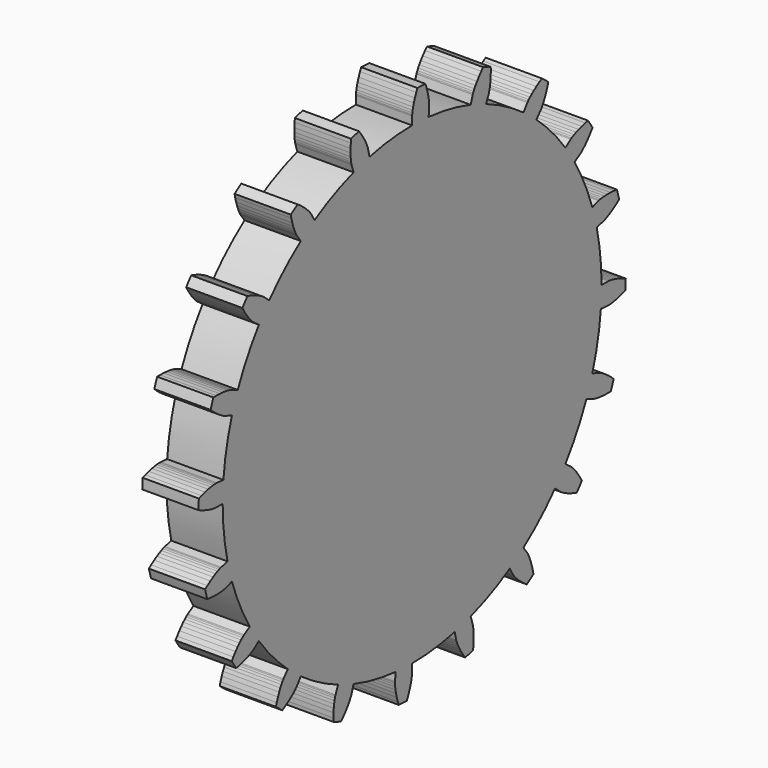
from build123d import *

# Parameters (mm, degrees)
F2_DEPTH = 6.35


# Not quite as in the source:
# - a variable given as a bare number and used for a length is read in inches; the dataset says mm whatever the document's units were


with BuildPart() as f2:
    # F1 (on Right) → F2 (new body)
    with BuildSketch(Plane.YZ):
        with BuildLine():
            ThreePointArc((26.6365153387, -2.330393128), (26.7128135988, -1.1663066295), (26.7382625, 0))
            ThreePointArc((26.7382625, 0), (26.5663850897, 3.0268572456), (26.0529625644, 6.0148003407))
            ThreePointArc((26.0529625644, 6.0148003407), (25.7658040109, 7.1454898497), (25.429598785, 8.2625775126))
            ThreePointArc((25.429598785, 8.2625775126), (24.3307833255, 11.0881767791), (22.9191642926, 13.7712232444))
            ThreePointArc((22.9191642926, 13.7712232444), (22.2966580055, 14.7578359967), (21.6317087626, 15.7163563694))
            ThreePointArc((21.6317087626, 15.7163563694), (19.7135149669, 18.0641083137), (17.5418785326, 20.1796228673))
            ThreePointArc((17.5418785326, 20.1796228673), (16.6449597645, 20.9255823326), (15.7163563694, 21.6317087626))
            ThreePointArc((15.7163563694, 21.6317087626), (13.1665504112, 23.2717990664), (10.4474714805, 24.6127004041))
            ThreePointArc((10.4474714805, 24.6127004041), (9.3639368896, 25.0449868726), (8.2625775126, 25.429598785))
            ThreePointArc((8.2625775126, 25.429598785), (5.3307521645, 26.2014839824), (2.330393128, 26.6365153387))
            ThreePointArc((2.330393128, 26.6365153387), (1.1663066295, 26.7128135988), (0, 26.7382625))
            ThreePointArc((0, 26.7382625), (-3.0268572456, 26.5663850897), (-6.0148003407, 26.0529625644))
            ThreePointArc((-6.0148003407, 26.0529625644), (-7.1454898497, 25.7658040109), (-8.2625775126, 25.429598785))
            ThreePointArc((-8.2625775126, 25.429598785), (-11.0881767791, 24.3307833255), (-13.7712232444, 22.9191642926))
            ThreePointArc((-13.7712232444, 22.9191642926), (-14.7578359967, 22.2966580055), (-15.7163563694, 21.6317087626))
            ThreePointArc((-15.7163563694, 21.6317087626), (-18.0641083137, 19.7135149669), (-20.1796228673, 17.5418785326))
            ThreePointArc((-20.1796228673, 17.5418785326), (-20.9255823326, 16.6449597645), (-21.6317087626, 15.7163563694))
            ThreePointArc((-21.6317087626, 15.7163563694), (-23.2717990664, 13.1665504112), (-24.6127004041, 10.4474714805))
            ThreePointArc((-24.6127004041, 10.4474714805), (-25.0449868726, 9.3639368896), (-25.429598785, 8.2625775126))
            ThreePointArc((-25.429598785, 8.2625775126), (-26.2014839824, 5.3307521645), (-26.6365153387, 2.330393128))
            ThreePointArc((-26.6365153387, 2.330393128), (-26.7128135988, 1.1663066295), (-26.7382625, 0))
            ThreePointArc((-26.7382625, 0), (-26.5663850897, -3.0268572456), (-26.0529625644, -6.0148003407))
            ThreePointArc((-26.0529625644, -6.0148003407), (-25.7658040109, -7.1454898497), (-25.429598785, -8.2625775126))
            ThreePointArc((-25.429598785, -8.2625775126), (-24.3307833255, -11.0881767791), (-22.9191642926, -13.7712232444))
            ThreePointArc((-22.9191642926, -13.7712232444), (-22.2966580055, -14.7578359967), (-21.6317087626, -15.7163563694))
            ThreePointArc((-21.6317087626, -15.7163563694), (-19.7135149669, -18.0641083137), (-17.5418785326, -20.1796228673))
            ThreePointArc((-17.5418785326, -20.1796228673), (-16.6449597645, -20.9255823326), (-15.7163563694, -21.6317087626))
            ThreePointArc((-15.7163563694, -21.6317087626), (-13.1665504112, -23.2717990664), (-10.4474714805, -24.6127004041))
            ThreePointArc((-10.4474714805, -24.6127004041), (-9.3639368896, -25.0449868726), (-8.2625775126, -25.429598785))
            ThreePointArc((-8.2625775126, -25.429598785), (-5.3307521645, -26.2014839824), (-2.330393128, -26.6365153387))
            ThreePointArc((-2.330393128, -26.6365153387), (-1.1663066295, -26.7128135988), (0, -26.7382625))
            ThreePointArc((0, -26.7382625), (3.0268572456, -26.5663850897), (6.0148003407, -26.0529625644))
            ThreePointArc((6.0148003407, -26.0529625644), (7.1454898497, -25.7658040109), (8.2625775126, -25.429598785))
            ThreePointArc((8.2625775126, -25.429598785), (11.0881767791, -24.3307833255), (13.7712232444, -22.9191642926))
            ThreePointArc((13.7712232444, -22.9191642926), (14.7578359967, -22.2966580055), (15.7163563694, -21.6317087626))
            ThreePointArc((15.7163563694, -21.6317087626), (18.0641083137, -19.7135149669), (20.1796228673, -17.5418785326))
            ThreePointArc((20.1796228673, -17.5418785326), (20.9255823326, -16.6449597645), (21.6317087626, -15.7163563694))
            ThreePointArc((21.6317087626, -15.7163563694), (23.2717990664, -13.1665504112), (24.6127004041, -10.4474714805))
            ThreePointArc((24.6127004041, -10.4474714805), (25.0449868726, -9.3639368896), (25.429598785, -8.2625775126))
            ThreePointArc((25.429598785, -8.2625775126), (26.2014839824, -5.3307521645), (26.6365153387, -2.330393128))
        make_face()
        with BuildLine():
            Line((-26.3108062145, -8.5488991629), (-25.429598785, -8.2625775126))
            ThreePointArc((-25.429598785, -8.2625775126), (-25.7658040109, -7.1454898497), (-26.0529625644, -6.0148003407))
            Line((-26.0529625644, -6.0148003407), (-26.9557713096, -6.2232301626))
            Line((-26.9557713096, -6.2232301626), (-26.9891857357, -6.2321271956))
            Line((-26.9891857357, -6.2321271956), (-27.088141079, -6.2632448013))
            Line((-27.088141079, -6.2632448013), (-27.250334693, -6.3231051855))
            Line((-27.250334693, -6.3231051855), (-27.4729785748, -6.4180477409))
            Line((-27.4729785748, -6.4180477409), (-27.7528122899, -6.5541969827))
            Line((-27.7528122899, -6.5541969827), (-28.0861178795, -6.73743134))
            Line((-28.0861178795, -6.73743134), (-28.4687366983, -6.9733529183))
            Line((-28.4687366983, -6.9733529183), (-28.8960881212, -7.2672583507))
            Line((-28.8960881212, -7.2672583507), (-29.2128054383, -7.5092213093))
            ThreePointArc((-29.2128054383, -7.5092213093), (-29.0655035449, -8.0605775185), (-28.9077964707, -8.6090481156))
            Line((-28.9077964707, -8.6090481156), (-28.5116966065, -8.6533293744))
            Line((-28.5116966065, -8.6533293744), (-27.9940124528, -8.6851532464))
            Line((-27.9940124528, -8.6851532464), (-27.5445355172, -8.690314249))
            Line((-27.5445355172, -8.690314249), (-27.164464194, -8.6757116792))
            Line((-27.164464194, -8.6757116792), (-26.8544778404, -8.6482893394))
            Line((-26.8544778404, -8.6482893394), (-26.6147357542, -8.615000917))
            Line((-26.6147357542, -8.615000917), (-26.4448783149, -8.5827753943))
            Line((-26.4448783149, -8.5827753943), (-26.3440302786, -8.5584826188))
            Line((-26.3440302786, -8.5584826188), (-26.3108062145, -8.5488991629))
        make_face()
        with BuildLine():
            Line((-22.3813085748, -16.260972512), (-21.6317087626, -15.7163563694))
            ThreePointArc((-21.6317087626, -15.7163563694), (-22.2966580055, -14.7578359967), (-22.9191642926, -13.7712232444))
            Line((-22.9191642926, -13.7712232444), (-23.7133780756, -14.2484350297))
            Line((-23.7133780756, -14.2484350297), (-23.7424077489, -14.2672222364))
            Line((-23.7424077489, -14.2672222364), (-23.826904004, -14.3273957209))
            Line((-23.826904004, -14.3273957209), (-23.9626614214, -14.4344469125))
            Line((-23.9626614214, -14.4344469125), (-24.145069473, -14.5935433916))
            Line((-24.145069473, -14.5935433916), (-24.3691347217, -14.8095023888))
            Line((-24.3691347217, -14.8095023888), (-24.6295046443, -15.0867657098))
            Line((-24.6295046443, -15.0867657098), (-24.9204929881, -15.4293761816))
            Line((-24.9204929881, -15.4293761816), (-25.2361065702, -15.8409557104))
            Line((-25.2361065702, -15.8409557104), (-25.4625519723, -16.1689471923))
            ThreePointArc((-25.4625519723, -16.1689471923), (-25.1520811081, -16.6477993195), (-24.8326060321, -17.1206916888))
            Line((-24.8326060321, -17.1206916888), (-24.4422090136, -17.040404079))
            Line((-24.4422090136, -17.040404079), (-23.9400280086, -16.9106971787))
            Line((-23.9400280086, -16.9106971787), (-23.5109552026, -16.7767095721))
            Line((-23.5109552026, -16.7767095721), (-23.1539983362, -16.645373205))
            Line((-23.1539983362, -16.645373205), (-22.8676577636, -16.5235019588))
            Line((-22.8676577636, -16.5235019588), (-22.6499361786, -16.4177584088))
            Line((-22.6499361786, -16.4177584088), (-22.4983503883, -16.3346212801))
            Line((-22.4983503883, -16.3346212801), (-22.4099450866, -16.2803537206))
            Line((-22.4099450866, -16.2803537206), (-22.3813085748, -16.260972512))
        make_face()
        with BuildLine():
            Line((-16.260972512, -22.3813085748), (-15.7163563694, -21.6317087626))
            ThreePointArc((-15.7163563694, -21.6317087626), (-16.6449597645, -20.9255823326), (-17.5418785326, -20.1796228673))
            Line((-17.5418785326, -20.1796228673), (-18.1497541747, -20.8789038015))
            Line((-18.1497541747, -20.8789038015), (-18.1715574685, -20.9057421591))
            Line((-18.1715574685, -20.9057421591), (-18.2333235533, -20.9890813225))
            Line((-18.2333235533, -20.9890813225), (-18.3293558923, -21.1328444049))
            Line((-18.3293558923, -21.1328444049), (-18.4536727425, -21.3405213359))
            Line((-18.4536727425, -21.3405213359), (-18.6000364572, -21.6151505172))
            Line((-18.6000364572, -21.6151505172), (-18.7619838906, -21.9593023362))
            Line((-18.7619838906, -21.9593023362), (-18.9328577929, -22.3750646014))
            Line((-18.9328577929, -22.3750646014), (-19.1058390779, -22.8640299548))
            Line((-19.1058390779, -22.8640299548), (-19.2198465112, -23.2459438685))
            ThreePointArc((-19.2198465112, -23.2459438685), (-18.7765977276, -23.6054185311), (-18.3266270961, -23.9564426727))
            Line((-18.3266270961, -23.9564426727), (-17.9801477036, -23.7594453049))
            Line((-17.9801477036, -23.7594453049), (-17.5426268229, -23.4809042473))
            Line((-17.5426268229, -23.4809042473), (-17.1759587822, -23.2208836721))
            Line((-17.1759587822, -23.2208836721), (-16.8770577979, -22.9856696264))
            Line((-16.8770577979, -22.9856696264), (-16.6423920167, -22.7812790804))
            Line((-16.6423920167, -22.7812790804), (-16.4680030385, -22.6134313184))
            Line((-16.4680030385, -22.6134313184), (-16.3495271705, -22.487520625))
            Line((-16.3495271705, -22.487520625), (-16.2822183303, -22.4085903684))
            Line((-16.2822183303, -22.4085903684), (-16.260972512, -22.3813085748))
        make_face()
        with BuildLine():
            Line((-8.5488991629, -26.3108062145), (-8.2625775126, -25.429598785))
            ThreePointArc((-8.2625775126, -25.429598785), (-9.3639368896, -25.0449868726), (-10.4474714805, -24.6127004041))
            Line((-10.4474714805, -24.6127004041), (-10.8095058785, -25.4655999972))
            Line((-10.8095058785, -25.4655999972), (-10.8219485345, -25.4978623804))
            Line((-10.8219485345, -25.4978623804), (-10.8549383541, -25.5962094047))
            Line((-10.8549383541, -25.5962094047), (-10.9018453002, -25.7626118458))
            Line((-10.9018453002, -25.7626118458), (-10.9559019498, -25.9985403637))
            Line((-10.9559019498, -25.9985403637), (-11.0102370301, -26.3049571113))
            Line((-11.0102370301, -26.3049571113), (-11.0579094312, -26.6823094505))
            Line((-11.0579094312, -26.6823094505), (-11.091942564, -27.1305258017))
            Line((-11.091942564, -27.1305258017), (-11.1053589384, -27.6490136441))
            Line((-11.1053589384, -27.6490136441), (-11.095768561, -28.0474655948))
            ThreePointArc((-11.095768561, -28.0474655948), (-10.5631301372, -28.2523749082), (-10.0267102108, -28.4471701334))
            Line((-10.0267102108, -28.4471701334), (-9.7580642613, -28.1527464826))
            Line((-9.7580642613, -28.1527464826), (-9.4280310972, -27.7526368072))
            Line((-9.4280310972, -27.7526368072), (-9.1596598444, -27.3920358889))
            Line((-9.1596598444, -27.3920358889), (-8.9480732529, -27.0759685542))
            Line((-8.9480732529, -27.0759685542), (-8.7880529847, -26.8090658792))
            Line((-8.7880529847, -26.8090658792), (-8.6740670216, -26.5955440134))
            Line((-8.6740670216, -26.5955440134), (-8.6002983193, -26.4391847714))
            Line((-8.6002983193, -26.4391847714), (-8.560674599, -26.343318061))
            Line((-8.560674599, -26.343318061), (-8.5488991629, -26.3108062145))
        make_face()
        with BuildLine():
            Line((0, -27.6648188238), (0, -26.7382625))
            ThreePointArc((0, -26.7382625), (-1.1663066295, -26.7128135988), (-2.330393128, -26.6365153387))
            Line((-2.330393128, -26.6365153387), (-2.4111478326, -27.5595458359))
            Line((-2.4111478326, -27.5595458359), (-2.4130118769, -27.5940741779))
            Line((-2.4130118769, -27.5940741779), (-2.413996158, -27.6978021711))
            Line((-2.413996158, -27.6978021711), (-2.4071861326, -27.8705553405))
            Line((-2.4071861326, -27.8705553405), (-2.3856911399, -28.1116411182))
            Line((-2.3856911399, -28.1116411182), (-2.3426788898, -28.419851226))
            Line((-2.3426788898, -28.419851226), (-2.2714097518, -28.7934662093))
            Line((-2.2714097518, -28.7934662093), (-2.1652707148, -29.2302621072))
            Line((-2.1652707148, -29.2302621072), (-2.0178088904, -29.727519236))
            Line((-2.0178088904, -29.727519236), (-1.8855594753, -30.1035059705))
            ThreePointArc((-1.8855594753, -30.1035059705), (-1.3156697714, -30.1337919835), (-0.7453090699, -30.1532903783))
            Line((-0.7453090699, -30.1532903783), (-0.5807935007, -29.7902606828))
            Line((-0.5807935007, -29.7902606828), (-0.3905539987, -29.3077479124))
            Line((-0.3905539987, -29.3077479124), (-0.2467495818, -28.8818647813))
            Line((-0.2467495818, -28.8818647813), (-0.1431889531, -28.5158830306))
            Line((-0.1431889531, -28.5158830306), (-0.0734780967, -28.2125945199))
            Line((-0.0734780967, -28.2125945199), (-0.0310528889, -27.9742995584))
            Line((-0.0310528889, -27.9742995584), (-0.0092123469, -27.8027972998))
            Line((-0.0092123469, -27.8027972998), (-0.0011523922, -27.6993782372))
            Line((-0.0011523922, -27.6993782372), (0, -27.6648188238))
        make_face()
        with BuildLine():
            Line((8.5488991629, -26.3108062145), (8.2625775126, -25.429598785))
            ThreePointArc((8.2625775126, -25.429598785), (7.1454898497, -25.7658040109), (6.0148003407, -26.0529625644))
            Line((6.0148003407, -26.0529625644), (6.2232301626, -26.9557713096))
            Line((6.2232301626, -26.9557713096), (6.2321271956, -26.9891857357))
            Line((6.2321271956, -26.9891857357), (6.2632448013, -27.088141079))
            Line((6.2632448013, -27.088141079), (6.3231051855, -27.250334693))
            Line((6.3231051855, -27.250334693), (6.4180477409, -27.4729785748))
            Line((6.4180477409, -27.4729785748), (6.5541969827, -27.7528122899))
            Line((6.5541969827, -27.7528122899), (6.73743134, -28.0861178795))
            Line((6.73743134, -28.0861178795), (6.9733529183, -28.4687366983))
            Line((6.9733529183, -28.4687366983), (7.2672583507, -28.8960881212))
            Line((7.2672583507, -28.8960881212), (7.5092213093, -29.2128054383))
            ThreePointArc((7.5092213093, -29.2128054383), (8.0605775185, -29.0655035449), (8.6090481156, -28.9077964707))
            Line((8.6090481156, -28.9077964707), (8.6533293744, -28.5116966065))
            Line((8.6533293744, -28.5116966065), (8.6851532464, -27.9940124528))
            Line((8.6851532464, -27.9940124528), (8.690314249, -27.5445355172))
            Line((8.690314249, -27.5445355172), (8.6757116792, -27.164464194))
            Line((8.6757116792, -27.164464194), (8.6482893394, -26.8544778404))
            Line((8.6482893394, -26.8544778404), (8.615000917, -26.6147357542))
            Line((8.615000917, -26.6147357542), (8.5827753943, -26.4448783149))
            Line((8.5827753943, -26.4448783149), (8.5584826188, -26.3440302786))
            Line((8.5584826188, -26.3440302786), (8.5488991629, -26.3108062145))
        make_face()
        with BuildLine():
            Line((16.260972512, -22.3813085748), (15.7163563694, -21.6317087626))
            ThreePointArc((15.7163563694, -21.6317087626), (14.7578359967, -22.2966580055), (13.7712232444, -22.9191642926))
            Line((13.7712232444, -22.9191642926), (14.2484350297, -23.7133780756))
            Line((14.2484350297, -23.7133780756), (14.2672222364, -23.7424077489))
            Line((14.2672222364, -23.7424077489), (14.3273957209, -23.826904004))
            Line((14.3273957209, -23.826904004), (14.4344469125, -23.9626614214))
            Line((14.4344469125, -23.9626614214), (14.5935433916, -24.145069473))
            Line((14.5935433916, -24.145069473), (14.8095023888, -24.3691347217))
            Line((14.8095023888, -24.3691347217), (15.0867657098, -24.6295046443))
            Line((15.0867657098, -24.6295046443), (15.4293761816, -24.9204929881))
            Line((15.4293761816, -24.9204929881), (15.8409557104, -25.2361065702))
            Line((15.8409557104, -25.2361065702), (16.1689471923, -25.4625519723))
            ThreePointArc((16.1689471923, -25.4625519723), (16.6477993195, -25.1520811081), (17.1206916888, -24.8326060321))
            Line((17.1206916888, -24.8326060321), (17.040404079, -24.4422090136))
            Line((17.040404079, -24.4422090136), (16.9106971787, -23.9400280086))
            Line((16.9106971787, -23.9400280086), (16.7767095721, -23.5109552026))
            Line((16.7767095721, -23.5109552026), (16.645373205, -23.1539983362))
            Line((16.645373205, -23.1539983362), (16.5235019588, -22.8676577636))
            Line((16.5235019588, -22.8676577636), (16.4177584088, -22.6499361786))
            Line((16.4177584088, -22.6499361786), (16.3346212801, -22.4983503883))
            Line((16.3346212801, -22.4983503883), (16.2803537206, -22.4099450866))
            Line((16.2803537206, -22.4099450866), (16.260972512, -22.3813085748))
        make_face()
        with BuildLine():
            Line((22.3813085748, -16.260972512), (21.6317087626, -15.7163563694))
            ThreePointArc((21.6317087626, -15.7163563694), (20.9255823326, -16.6449597645), (20.1796228673, -17.5418785326))
            Line((20.1796228673, -17.5418785326), (20.8789038015, -18.1497541747))
            Line((20.8789038015, -18.1497541747), (20.9057421591, -18.1715574685))
            Line((20.9057421591, -18.1715574685), (20.9890813225, -18.2333235533))
            Line((20.9890813225, -18.2333235533), (21.1328444049, -18.3293558923))
            Line((21.1328444049, -18.3293558923), (21.3405213359, -18.4536727425))
            Line((21.3405213359, -18.4536727425), (21.6151505172, -18.6000364572))
            Line((21.6151505172, -18.6000364572), (21.9593023362, -18.7619838906))
            Line((21.9593023362, -18.7619838906), (22.3750646014, -18.9328577929))
            Line((22.3750646014, -18.9328577929), (22.8640299548, -19.1058390779))
            Line((22.8640299548, -19.1058390779), (23.2459438685, -19.2198465112))
            ThreePointArc((23.2459438685, -19.2198465112), (23.6054185311, -18.7765977276), (23.9564426727, -18.3266270961))
            Line((23.9564426727, -18.3266270961), (23.7594453049, -17.9801477036))
            Line((23.7594453049, -17.9801477036), (23.4809042473, -17.5426268229))
            Line((23.4809042473, -17.5426268229), (23.2208836721, -17.1759587822))
            Line((23.2208836721, -17.1759587822), (22.9856696264, -16.8770577979))
            Line((22.9856696264, -16.8770577979), (22.7812790804, -16.6423920167))
            Line((22.7812790804, -16.6423920167), (22.6134313184, -16.4680030385))
            Line((22.6134313184, -16.4680030385), (22.487520625, -16.3495271705))
            Line((22.487520625, -16.3495271705), (22.4085903684, -16.2822183303))
            Line((22.4085903684, -16.2822183303), (22.3813085748, -16.260972512))
        make_face()
        with BuildLine():
            Line((26.3108062145, -8.5488991629), (25.429598785, -8.2625775126))
            ThreePointArc((25.429598785, -8.2625775126), (25.0449868726, -9.3639368896), (24.6127004041, -10.4474714805))
            Line((24.6127004041, -10.4474714805), (25.4655999972, -10.8095058785))
            Line((25.4655999972, -10.8095058785), (25.4978623804, -10.8219485345))
            Line((25.4978623804, -10.8219485345), (25.5962094047, -10.8549383541))
            Line((25.5962094047, -10.8549383541), (25.7626118458, -10.9018453002))
            Line((25.7626118458, -10.9018453002), (25.9985403637, -10.9559019498))
            Line((25.9985403637, -10.9559019498), (26.3049571113, -11.0102370301))
            Line((26.3049571113, -11.0102370301), (26.6823094505, -11.0579094312))
            Line((26.6823094505, -11.0579094312), (27.1305258017, -11.091942564))
            Line((27.1305258017, -11.091942564), (27.6490136441, -11.1053589384))
            Line((27.6490136441, -11.1053589384), (28.0474655948, -11.095768561))
            ThreePointArc((28.0474655948, -11.095768561), (28.2523749082, -10.5631301372), (28.4471701334, -10.0267102108))
            Line((28.4471701334, -10.0267102108), (28.1527464826, -9.7580642613))
            Line((28.1527464826, -9.7580642613), (27.7526368072, -9.4280310972))
            Line((27.7526368072, -9.4280310972), (27.3920358889, -9.1596598444))
            Line((27.3920358889, -9.1596598444), (27.0759685542, -8.9480732529))
            Line((27.0759685542, -8.9480732529), (26.8090658792, -8.7880529847))
            Line((26.8090658792, -8.7880529847), (26.5955440134, -8.6740670216))
            Line((26.5955440134, -8.6740670216), (26.4391847714, -8.6002983193))
            Line((26.4391847714, -8.6002983193), (26.343318061, -8.560674599))
            Line((26.343318061, -8.560674599), (26.3108062145, -8.5488991629))
        make_face()
        with BuildLine():
            Line((27.6648188238, 0), (26.7382625, 0))
            ThreePointArc((26.7382625, 0), (26.7128135988, -1.1663066295), (26.6365153387, -2.330393128))
            Line((26.6365153387, -2.330393128), (27.5595458359, -2.4111478326))
            Line((27.5595458359, -2.4111478326), (27.5940741779, -2.4130118769))
            Line((27.5940741779, -2.4130118769), (27.6978021711, -2.413996158))
            Line((27.6978021711, -2.413996158), (27.8705553405, -2.4071861326))
            Line((27.8705553405, -2.4071861326), (28.1116411182, -2.3856911399))
            Line((28.1116411182, -2.3856911399), (28.419851226, -2.3426788898))
            Line((28.419851226, -2.3426788898), (28.7934662093, -2.2714097518))
            Line((28.7934662093, -2.2714097518), (29.2302621072, -2.1652707148))
            Line((29.2302621072, -2.1652707148), (29.727519236, -2.0178088904))
            Line((29.727519236, -2.0178088904), (30.1035059705, -1.8855594753))
            ThreePointArc((30.1035059705, -1.8855594753), (30.1337919835, -1.3156697714), (30.1532903783, -0.7453090699))
            Line((30.1532903783, -0.7453090699), (29.7902606828, -0.5807935007))
            Line((29.7902606828, -0.5807935007), (29.3077479124, -0.3905539987))
            Line((29.3077479124, -0.3905539987), (28.8818647813, -0.2467495818))
            Line((28.8818647813, -0.2467495818), (28.5158830306, -0.1431889531))
            Line((28.5158830306, -0.1431889531), (28.2125945199, -0.0734780967))
            Line((28.2125945199, -0.0734780967), (27.9742995584, -0.0310528889))
            Line((27.9742995584, -0.0310528889), (27.8027972998, -0.0092123469))
            Line((27.8027972998, -0.0092123469), (27.6993782372, -0.0011523922))
            Line((27.6993782372, -0.0011523922), (27.6648188238, 0))
        make_face()
        with BuildLine():
            ThreePointArc((25.429598785, 8.2625775126), (25.7658040109, 7.1454898497), (26.0529625644, 6.0148003407))
            Line((26.0529625644, 6.0148003407), (26.9557713096, 6.2232301626))
            Line((26.9557713096, 6.2232301626), (26.9891857357, 6.2321271956))
            Line((26.9891857357, 6.2321271956), (27.088141079, 6.2632448013))
            Line((27.088141079, 6.2632448013), (27.250334693, 6.3231051855))
            Line((27.250334693, 6.3231051855), (27.4729785748, 6.4180477409))
            Line((27.4729785748, 6.4180477409), (27.7528122899, 6.5541969827))
            Line((27.7528122899, 6.5541969827), (28.0861178795, 6.73743134))
            Line((28.0861178795, 6.73743134), (28.4687366983, 6.9733529183))
            Line((28.4687366983, 6.9733529183), (28.8960881212, 7.2672583507))
            Line((28.8960881212, 7.2672583507), (29.2128054383, 7.5092213093))
            ThreePointArc((29.2128054383, 7.5092213093), (29.0655035449, 8.0605775185), (28.9077964707, 8.6090481156))
            Line((28.9077964707, 8.6090481156), (28.5116966065, 8.6533293744))
            Line((28.5116966065, 8.6533293744), (27.9940124528, 8.6851532464))
            Line((27.9940124528, 8.6851532464), (27.5445355172, 8.690314249))
            Line((27.5445355172, 8.690314249), (27.164464194, 8.6757116792))
            Line((27.164464194, 8.6757116792), (26.8544778404, 8.6482893394))
            Line((26.8544778404, 8.6482893394), (26.6147357542, 8.615000917))
            Line((26.6147357542, 8.615000917), (26.4448783149, 8.5827753943))
            Line((26.4448783149, 8.5827753943), (26.3440302786, 8.5584826188))
            Line((26.3440302786, 8.5584826188), (26.3108062145, 8.5488991629))
            Line((26.3108062145, 8.5488991629), (25.429598785, 8.2625775126))
        make_face()
        with BuildLine():
            ThreePointArc((21.6317087626, 15.7163563694), (22.2966580055, 14.7578359967), (22.9191642926, 13.7712232444))
            Line((22.9191642926, 13.7712232444), (23.7133780756, 14.2484350297))
            Line((23.7133780756, 14.2484350297), (23.7424077489, 14.2672222364))
            Line((23.7424077489, 14.2672222364), (23.826904004, 14.3273957209))
            Line((23.826904004, 14.3273957209), (23.9626614214, 14.4344469125))
            Line((23.9626614214, 14.4344469125), (24.145069473, 14.5935433916))
            Line((24.145069473, 14.5935433916), (24.3691347217, 14.8095023888))
            Line((24.3691347217, 14.8095023888), (24.6295046443, 15.0867657098))
            Line((24.6295046443, 15.0867657098), (24.9204929881, 15.4293761816))
            Line((24.9204929881, 15.4293761816), (25.2361065702, 15.8409557104))
            Line((25.2361065702, 15.8409557104), (25.4625519723, 16.1689471923))
            ThreePointArc((25.4625519723, 16.1689471923), (25.1520811081, 16.6477993195), (24.8326060321, 17.1206916888))
            Line((24.8326060321, 17.1206916888), (24.4422090136, 17.040404079))
            Line((24.4422090136, 17.040404079), (23.9400280086, 16.9106971787))
            Line((23.9400280086, 16.9106971787), (23.5109552026, 16.7767095721))
            Line((23.5109552026, 16.7767095721), (23.1539983362, 16.645373205))
            Line((23.1539983362, 16.645373205), (22.8676577636, 16.5235019588))
            Line((22.8676577636, 16.5235019588), (22.6499361786, 16.4177584088))
            Line((22.6499361786, 16.4177584088), (22.4983503883, 16.3346212801))
            Line((22.4983503883, 16.3346212801), (22.4099450866, 16.2803537206))
            Line((22.4099450866, 16.2803537206), (22.3813085748, 16.260972512))
            Line((22.3813085748, 16.260972512), (21.6317087626, 15.7163563694))
        make_face()
        with BuildLine():
            ThreePointArc((15.7163563694, 21.6317087626), (16.6449597645, 20.9255823326), (17.5418785326, 20.1796228673))
            Line((17.5418785326, 20.1796228673), (18.1497541747, 20.8789038015))
            Line((18.1497541747, 20.8789038015), (18.1715574685, 20.9057421591))
            Line((18.1715574685, 20.9057421591), (18.2333235533, 20.9890813225))
            Line((18.2333235533, 20.9890813225), (18.3293558923, 21.1328444049))
            Line((18.3293558923, 21.1328444049), (18.4536727425, 21.3405213359))
            Line((18.4536727425, 21.3405213359), (18.6000364572, 21.6151505172))
            Line((18.6000364572, 21.6151505172), (18.7619838906, 21.9593023362))
            Line((18.7619838906, 21.9593023362), (18.9328577929, 22.3750646014))
            Line((18.9328577929, 22.3750646014), (19.1058390779, 22.8640299548))
            Line((19.1058390779, 22.8640299548), (19.2198465112, 23.2459438685))
            ThreePointArc((19.2198465112, 23.2459438685), (18.7765977276, 23.6054185311), (18.3266270961, 23.9564426727))
            Line((18.3266270961, 23.9564426727), (17.9801477036, 23.7594453049))
            Line((17.9801477036, 23.7594453049), (17.5426268229, 23.4809042473))
            Line((17.5426268229, 23.4809042473), (17.1759587822, 23.2208836721))
            Line((17.1759587822, 23.2208836721), (16.8770577979, 22.9856696264))
            Line((16.8770577979, 22.9856696264), (16.6423920167, 22.7812790804))
            Line((16.6423920167, 22.7812790804), (16.4680030385, 22.6134313184))
            Line((16.4680030385, 22.6134313184), (16.3495271705, 22.487520625))
            Line((16.3495271705, 22.487520625), (16.2822183303, 22.4085903684))
            Line((16.2822183303, 22.4085903684), (16.260972512, 22.3813085748))
            Line((16.260972512, 22.3813085748), (15.7163563694, 21.6317087626))
        make_face()
        with BuildLine():
            ThreePointArc((8.2625775126, 25.429598785), (9.3639368896, 25.0449868726), (10.4474714805, 24.6127004041))
            Line((10.4474714805, 24.6127004041), (10.8095058785, 25.4655999972))
            Line((10.8095058785, 25.4655999972), (10.8219485345, 25.4978623804))
            Line((10.8219485345, 25.4978623804), (10.8549383541, 25.5962094047))
            Line((10.8549383541, 25.5962094047), (10.9018453002, 25.7626118458))
            Line((10.9018453002, 25.7626118458), (10.9559019498, 25.9985403637))
            Line((10.9559019498, 25.9985403637), (11.0102370301, 26.3049571113))
            Line((11.0102370301, 26.3049571113), (11.0579094312, 26.6823094505))
            Line((11.0579094312, 26.6823094505), (11.091942564, 27.1305258017))
            Line((11.091942564, 27.1305258017), (11.1053589384, 27.6490136441))
            Line((11.1053589384, 27.6490136441), (11.095768561, 28.0474655948))
            ThreePointArc((11.095768561, 28.0474655948), (10.5631301372, 28.2523749082), (10.0267102108, 28.4471701334))
            Line((10.0267102108, 28.4471701334), (9.7580642613, 28.1527464826))
            Line((9.7580642613, 28.1527464826), (9.4280310972, 27.7526368072))
            Line((9.4280310972, 27.7526368072), (9.1596598444, 27.3920358889))
            Line((9.1596598444, 27.3920358889), (8.9480732529, 27.0759685542))
            Line((8.9480732529, 27.0759685542), (8.7880529847, 26.8090658792))
            Line((8.7880529847, 26.8090658792), (8.6740670216, 26.5955440134))
            Line((8.6740670216, 26.5955440134), (8.6002983193, 26.4391847714))
            Line((8.6002983193, 26.4391847714), (8.560674599, 26.343318061))
            Line((8.560674599, 26.343318061), (8.5488991629, 26.3108062145))
            Line((8.5488991629, 26.3108062145), (8.2625775126, 25.429598785))
        make_face()
        with BuildLine():
            ThreePointArc((0, 26.7382625), (1.1663066295, 26.7128135988), (2.330393128, 26.6365153387))
            Line((2.330393128, 26.6365153387), (2.4111478326, 27.5595458359))
            Line((2.4111478326, 27.5595458359), (2.4130118769, 27.5940741779))
            Line((2.4130118769, 27.5940741779), (2.413996158, 27.6978021711))
            Line((2.413996158, 27.6978021711), (2.4071861326, 27.8705553405))
            Line((2.4071861326, 27.8705553405), (2.3856911399, 28.1116411182))
            Line((2.3856911399, 28.1116411182), (2.3426788898, 28.419851226))
            Line((2.3426788898, 28.419851226), (2.2714097518, 28.7934662093))
            Line((2.2714097518, 28.7934662093), (2.1652707148, 29.2302621072))
            Line((2.1652707148, 29.2302621072), (2.0178088904, 29.727519236))
            Line((2.0178088904, 29.727519236), (1.8855594753, 30.1035059705))
            ThreePointArc((1.8855594753, 30.1035059705), (1.3156697714, 30.1337919835), (0.7453090699, 30.1532903783))
            Line((0.7453090699, 30.1532903783), (0.5807935007, 29.7902606828))
            Line((0.5807935007, 29.7902606828), (0.3905539987, 29.3077479124))
            Line((0.3905539987, 29.3077479124), (0.2467495818, 28.8818647813))
            Line((0.2467495818, 28.8818647813), (0.1431889531, 28.5158830306))
            Line((0.1431889531, 28.5158830306), (0.0734780967, 28.2125945199))
            Line((0.0734780967, 28.2125945199), (0.0310528889, 27.9742995584))
            Line((0.0310528889, 27.9742995584), (0.0092123469, 27.8027972998))
            Line((0.0092123469, 27.8027972998), (0.0011523922, 27.6993782372))
            Line((0.0011523922, 27.6993782372), (0, 27.6648188238))
            Line((0, 27.6648188238), (0, 26.7382625))
        make_face()
        with BuildLine():
            ThreePointArc((-8.2625775126, 25.429598785), (-7.1454898497, 25.7658040109), (-6.0148003407, 26.0529625644))
            Line((-6.0148003407, 26.0529625644), (-6.2232301626, 26.9557713096))
            Line((-6.2232301626, 26.9557713096), (-6.2321271956, 26.9891857357))
            Line((-6.2321271956, 26.9891857357), (-6.2632448013, 27.088141079))
            Line((-6.2632448013, 27.088141079), (-6.3231051855, 27.250334693))
            Line((-6.3231051855, 27.250334693), (-6.4180477409, 27.4729785748))
            Line((-6.4180477409, 27.4729785748), (-6.5541969827, 27.7528122899))
            Line((-6.5541969827, 27.7528122899), (-6.73743134, 28.0861178795))
            Line((-6.73743134, 28.0861178795), (-6.9733529183, 28.4687366983))
            Line((-6.9733529183, 28.4687366983), (-7.2672583507, 28.8960881212))
            Line((-7.2672583507, 28.8960881212), (-7.5092213093, 29.2128054383))
            ThreePointArc((-7.5092213093, 29.2128054383), (-8.0605775185, 29.0655035449), (-8.6090481156, 28.9077964707))
            Line((-8.6090481156, 28.9077964707), (-8.6533293744, 28.5116966065))
            Line((-8.6533293744, 28.5116966065), (-8.6851532464, 27.9940124528))
            Line((-8.6851532464, 27.9940124528), (-8.690314249, 27.5445355172))
            Line((-8.690314249, 27.5445355172), (-8.6757116792, 27.164464194))
            Line((-8.6757116792, 27.164464194), (-8.6482893394, 26.8544778404))
            Line((-8.6482893394, 26.8544778404), (-8.615000917, 26.6147357542))
            Line((-8.615000917, 26.6147357542), (-8.5827753943, 26.4448783149))
            Line((-8.5827753943, 26.4448783149), (-8.5584826188, 26.3440302786))
            Line((-8.5584826188, 26.3440302786), (-8.5488991629, 26.3108062145))
            Line((-8.5488991629, 26.3108062145), (-8.2625775126, 25.429598785))
        make_face()
        with BuildLine():
            ThreePointArc((-15.7163563694, 21.6317087626), (-14.7578359967, 22.2966580055), (-13.7712232444, 22.9191642926))
            Line((-13.7712232444, 22.9191642926), (-14.2484350297, 23.7133780756))
            Line((-14.2484350297, 23.7133780756), (-14.2672222364, 23.7424077489))
            Line((-14.2672222364, 23.7424077489), (-14.3273957209, 23.826904004))
            Line((-14.3273957209, 23.826904004), (-14.4344469125, 23.9626614214))
            Line((-14.4344469125, 23.9626614214), (-14.5935433916, 24.145069473))
            Line((-14.5935433916, 24.145069473), (-14.8095023888, 24.3691347217))
            Line((-14.8095023888, 24.3691347217), (-15.0867657098, 24.6295046443))
            Line((-15.0867657098, 24.6295046443), (-15.4293761816, 24.9204929881))
            Line((-15.4293761816, 24.9204929881), (-15.8409557104, 25.2361065702))
            Line((-15.8409557104, 25.2361065702), (-16.1689471923, 25.4625519723))
            ThreePointArc((-16.1689471923, 25.4625519723), (-16.6477993195, 25.1520811081), (-17.1206916888, 24.8326060321))
            Line((-17.1206916888, 24.8326060321), (-17.040404079, 24.4422090136))
            Line((-17.040404079, 24.4422090136), (-16.9106971787, 23.9400280086))
            Line((-16.9106971787, 23.9400280086), (-16.7767095721, 23.5109552026))
            Line((-16.7767095721, 23.5109552026), (-16.645373205, 23.1539983362))
            Line((-16.645373205, 23.1539983362), (-16.5235019588, 22.8676577636))
            Line((-16.5235019588, 22.8676577636), (-16.4177584088, 22.6499361786))
            Line((-16.4177584088, 22.6499361786), (-16.3346212801, 22.4983503883))
            Line((-16.3346212801, 22.4983503883), (-16.2803537206, 22.4099450866))
            Line((-16.2803537206, 22.4099450866), (-16.260972512, 22.3813085748))
            Line((-16.260972512, 22.3813085748), (-15.7163563694, 21.6317087626))
        make_face()
        with BuildLine():
            ThreePointArc((-21.6317087626, 15.7163563694), (-20.9255823326, 16.6449597645), (-20.1796228673, 17.5418785326))
            Line((-20.1796228673, 17.5418785326), (-20.8789038015, 18.1497541747))
            Line((-20.8789038015, 18.1497541747), (-20.9057421591, 18.1715574685))
            Line((-20.9057421591, 18.1715574685), (-20.9890813225, 18.2333235533))
            Line((-20.9890813225, 18.2333235533), (-21.1328444049, 18.3293558923))
            Line((-21.1328444049, 18.3293558923), (-21.3405213359, 18.4536727425))
            Line((-21.3405213359, 18.4536727425), (-21.6151505172, 18.6000364572))
            Line((-21.6151505172, 18.6000364572), (-21.9593023362, 18.7619838906))
            Line((-21.9593023362, 18.7619838906), (-22.3750646014, 18.9328577929))
            Line((-22.3750646014, 18.9328577929), (-22.8640299548, 19.1058390779))
            Line((-22.8640299548, 19.1058390779), (-23.2459438685, 19.2198465112))
            ThreePointArc((-23.2459438685, 19.2198465112), (-23.6054185311, 18.7765977276), (-23.9564426727, 18.3266270961))
            Line((-23.9564426727, 18.3266270961), (-23.7594453049, 17.9801477036))
            Line((-23.7594453049, 17.9801477036), (-23.4809042473, 17.5426268229))
            Line((-23.4809042473, 17.5426268229), (-23.2208836721, 17.1759587822))
            Line((-23.2208836721, 17.1759587822), (-22.9856696264, 16.8770577979))
            Line((-22.9856696264, 16.8770577979), (-22.7812790804, 16.6423920167))
            Line((-22.7812790804, 16.6423920167), (-22.6134313184, 16.4680030385))
            Line((-22.6134313184, 16.4680030385), (-22.487520625, 16.3495271705))
            Line((-22.487520625, 16.3495271705), (-22.4085903684, 16.2822183303))
            Line((-22.4085903684, 16.2822183303), (-22.3813085748, 16.260972512))
            Line((-22.3813085748, 16.260972512), (-21.6317087626, 15.7163563694))
        make_face()
        with BuildLine():
            ThreePointArc((-25.429598785, 8.2625775126), (-25.0449868726, 9.3639368896), (-24.6127004041, 10.4474714805))
            Line((-24.6127004041, 10.4474714805), (-25.4655999972, 10.8095058785))
            Line((-25.4655999972, 10.8095058785), (-25.4978623804, 10.8219485345))
            Line((-25.4978623804, 10.8219485345), (-25.5962094047, 10.8549383541))
            Line((-25.5962094047, 10.8549383541), (-25.7626118458, 10.9018453002))
            Line((-25.7626118458, 10.9018453002), (-25.9985403637, 10.9559019498))
            Line((-25.9985403637, 10.9559019498), (-26.3049571113, 11.0102370301))
            Line((-26.3049571113, 11.0102370301), (-26.6823094505, 11.0579094312))
            Line((-26.6823094505, 11.0579094312), (-27.1305258017, 11.091942564))
            Line((-27.1305258017, 11.091942564), (-27.6490136441, 11.1053589384))
            Line((-27.6490136441, 11.1053589384), (-28.0474655948, 11.095768561))
            ThreePointArc((-28.0474655948, 11.095768561), (-28.2523749082, 10.5631301372), (-28.4471701334, 10.0267102108))
            Line((-28.4471701334, 10.0267102108), (-28.1527464826, 9.7580642613))
            Line((-28.1527464826, 9.7580642613), (-27.7526368072, 9.4280310972))
            Line((-27.7526368072, 9.4280310972), (-27.3920358889, 9.1596598444))
            Line((-27.3920358889, 9.1596598444), (-27.0759685542, 8.9480732529))
            Line((-27.0759685542, 8.9480732529), (-26.8090658792, 8.7880529847))
            Line((-26.8090658792, 8.7880529847), (-26.5955440134, 8.6740670216))
            Line((-26.5955440134, 8.6740670216), (-26.4391847714, 8.6002983193))
            Line((-26.4391847714, 8.6002983193), (-26.343318061, 8.560674599))
            Line((-26.343318061, 8.560674599), (-26.3108062145, 8.5488991629))
            Line((-26.3108062145, 8.5488991629), (-25.429598785, 8.2625775126))
        make_face()
        with BuildLine():
            ThreePointArc((-26.7382625, 0), (-26.7128135988, 1.1663066295), (-26.6365153387, 2.330393128))
            Line((-26.6365153387, 2.330393128), (-27.5595458359, 2.4111478326))
            Line((-27.5595458359, 2.4111478326), (-27.5940741779, 2.4130118769))
            Line((-27.5940741779, 2.4130118769), (-27.6978021711, 2.413996158))
            Line((-27.6978021711, 2.413996158), (-27.8705553405, 2.4071861326))
            Line((-27.8705553405, 2.4071861326), (-28.1116411182, 2.3856911399))
            Line((-28.1116411182, 2.3856911399), (-28.419851226, 2.3426788898))
            Line((-28.419851226, 2.3426788898), (-28.7934662093, 2.2714097518))
            Line((-28.7934662093, 2.2714097518), (-29.2302621072, 2.1652707148))
            Line((-29.2302621072, 2.1652707148), (-29.727519236, 2.0178088904))
            Line((-29.727519236, 2.0178088904), (-30.1035059705, 1.8855594753))
            ThreePointArc((-30.1035059705, 1.8855594753), (-30.1337919835, 1.3156697714), (-30.1532903783, 0.7453090699))
            Line((-30.1532903783, 0.7453090699), (-29.7902606828, 0.5807935007))
            Line((-29.7902606828, 0.5807935007), (-29.3077479124, 0.3905539987))
            Line((-29.3077479124, 0.3905539987), (-28.8818647813, 0.2467495818))
            Line((-28.8818647813, 0.2467495818), (-28.5158830306, 0.1431889531))
            Line((-28.5158830306, 0.1431889531), (-28.2125945199, 0.0734780967))
            Line((-28.2125945199, 0.0734780967), (-27.9742995584, 0.0310528889))
            Line((-27.9742995584, 0.0310528889), (-27.8027972998, 0.0092123469))
            Line((-27.8027972998, 0.0092123469), (-27.6993782372, 0.0011523922))
            Line((-27.6993782372, 0.0011523922), (-27.6648188238, 0))
            Line((-27.6648188238, 0), (-26.7382625, 0))
        make_face()
    extrude(amount=F2_DEPTH)


solid = f2.part
